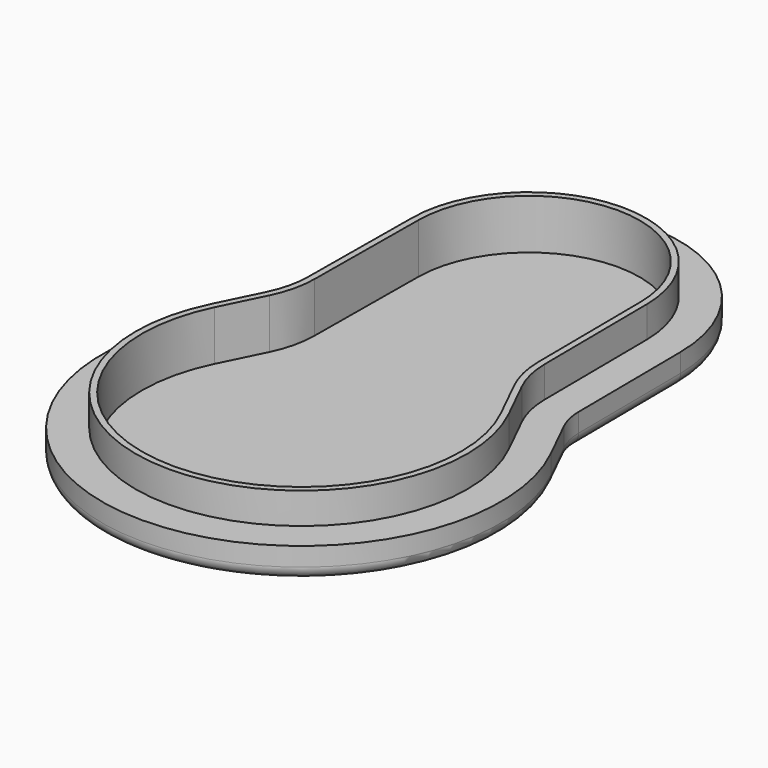
from build123d import *

# Parameters (mm, degrees)
F2_DEPTH = 4
F4_DEPTH = 1
F5_R     = 0.99999
F7_DEPTH = 1.5


# Not quite as in the source:
# - a fillet or chamfer is up to 0.001 mm smaller than in the source, because OpenCascade refuses the exact size


with BuildPart() as f2:
    # F1 (on face) → F2 (new body)
    with BuildSketch(Plane.XY):
        with BuildLine():
            ThreePointArc((-9.4849269336, 12.5314274341), (-9.6870039278, 10.8628934269), (-10.2555653995, 9.2812554476))
            Line((-10.2555653995, 9.2812554476), (-11.9329496797, 5.8732198956))
            ThreePointArc((-11.9329496797, 5.8732198956), (0, -13.3), (11.9329496797, 5.8732198956))
            Line((11.9329496797, 5.8732198956), (10.2555653995, 9.2812554476))
            ThreePointArc((10.2555653995, 9.2812554476), (9.6870039278, 10.8628934269), (9.4849269336, 12.5314274341))
            Line((9.4849269336, 12.5314274341), (9.3996809366, 22.8774486305))
            ThreePointArc((9.3996809366, 22.8774486305), (0, 32.2), (-9.3996809366, 22.8774486305))
            Line((-9.3996809366, 22.8774486305), (-9.4849269336, 12.5314274341))
        make_face()
        with BuildLine():
            ThreePointArc((-9.8069582687, 9.0604577072), (-9.2004926988, 10.7475382184), (-8.9849439051, 12.5273078261))
            Line((-8.9849439051, 12.5273078261), (-8.899697908, 22.8733290225))
            ThreePointArc((-8.899697908, 22.8733290225), (0, 31.7), (8.899697908, 22.8733290225))
            Line((8.899697908, 22.8733290225), (8.9849439051, 12.5273078261))
            ThreePointArc((8.9849439051, 12.5273078261), (9.2004926988, 10.7475382184), (9.8069582687, 9.0604577072))
            Line((9.8069582687, 9.0604577072), (11.4843425489, 5.6524221551))
            ThreePointArc((11.4843425489, 5.6524221551), (0, -12.8), (-11.4843425489, 5.6524221551))
            Line((-11.4843425489, 5.6524221551), (-9.8069582687, 9.0604577072))
        make_face(mode=Mode.SUBTRACT)
    extrude(amount=F2_DEPTH)

    # F3 (on face) + F0 (on Top) → F4 (join)
    with BuildSketch(Plane.XY):
        with BuildLine():
            ThreePointArc((12.6780439059, 10.473563246), (12.314164564, 11.4858115527), (12.1848352877, 12.5536733173))
            Line((12.1848352877, 12.5536733173), (12.0995892907, 22.8996945138))
            ThreePointArc((12.0995892907, 22.8996945138), (0, 34.9), (-12.0995892907, 22.8996945138))
            Line((-12.0995892907, 22.8996945138), (-12.1848352877, 12.5536733173))
            ThreePointArc((-12.1848352877, 12.5536733173), (-12.314164564, 11.4858115527), (-12.6780439059, 10.473563246))
            Line((-12.6780439059, 10.473563246), (-14.3554281861, 7.0655276939))
            ThreePointArc((-14.3554281861, 7.0655276939), (0, -16), (14.3554281861, 7.0655276939))
            Line((14.3554281861, 7.0655276939), (12.6780439059, 10.473563246))
        make_face()
        with BuildLine():
            ThreePointArc((-8.899697908, 22.8733290225), (0, 31.7), (8.899697908, 22.8733290225))
            Line((8.899697908, 22.8733290225), (8.9849439051, 12.5273078261))
            ThreePointArc((8.9849439051, 12.5273078261), (9.2004926988, 10.7475382184), (9.8069582687, 9.0604577072))
            Line((9.8069582687, 9.0604577072), (11.4843425489, 5.6524221551))
            ThreePointArc((11.4843425489, 5.6524221551), (0, -12.8), (-11.4843425489, 5.6524221551))
            Line((-11.4843425489, 5.6524221551), (-9.8069582687, 9.0604577072))
            ThreePointArc((-9.8069582687, 9.0604577072), (-9.2004926988, 10.7475382184), (-8.9849439051, 12.5273078261))
            Line((-8.9849439051, 12.5273078261), (-8.899697908, 22.8733290225))
        make_face(mode=Mode.SUBTRACT)
    with BuildSketch(Plane.XY):
        with BuildLine():
            Line((-9.8069582687, 9.0604577072), (-11.4843425489, 5.6524221551))
            ThreePointArc((-11.4843425489, 5.6524221551), (0, -12.8), (11.4843425489, 5.6524221551))
            Line((11.4843425489, 5.6524221551), (9.8069582687, 9.0604577072))
            ThreePointArc((9.8069582687, 9.0604577072), (9.2004926988, 10.7475382184), (8.9849439051, 12.5273078261))
            Line((8.9849439051, 12.5273078261), (8.899697908, 22.8733290225))
            ThreePointArc((8.899697908, 22.8733290225), (0, 31.7), (-8.899697908, 22.8733290225))
            Line((-8.899697908, 22.8733290225), (-8.9849439051, 12.5273078261))
            ThreePointArc((-8.9849439051, 12.5273078261), (-9.2004926988, 10.7475382184), (-9.8069582687, 9.0604577072))
        make_face()
    extrude(amount=-F4_DEPTH)

    # F5 (radius 1 in the source; OpenCascade refuses exactly that, so slightly less here)
    f5_edges = [f2.edges().sort_by_distance(p)[0] for p in [
        (0, -16, -1),
        (-13.516736, 8.769545, -1),
        (-12.314165, 11.485812, -1),
        (-12.142212, 17.726684, -1),
        (0, 34.9, -1),
        (12.142212, 17.726684, -1),
        (12.314165, 11.485812, -1),
        (13.516736, 8.769545, -1),
    ]]
    fillet(f5_edges, radius=F5_R)

    # F6 (on face) → F7 (join)
    with BuildSketch(Plane.XY):
        with BuildLine():
            ThreePointArc((-12.1848352877, 12.5536733173), (-12.314164564, 11.4858115527), (-12.6780439059, 10.473563246))
            Line((-12.6780439059, 10.473563246), (-14.3554281861, 7.0655276939))
            ThreePointArc((-14.3554281861, 7.0655276939), (0, -16), (14.3554281861, 7.0655276939))
            Line((14.3554281861, 7.0655276939), (12.6780439059, 10.473563246))
            ThreePointArc((12.6780439059, 10.473563246), (12.314164564, 11.4858115527), (12.1848352877, 12.5536733173))
            Line((12.1848352877, 12.5536733173), (12.0995892907, 22.8996945138))
            ThreePointArc((12.0995892907, 22.8996945138), (0, 34.9), (-12.0995892907, 22.8996945138))
            ThreePointArc((-12.0995892907, 22.8996945138), (-10.0273713078, 17.7092586924), (-12.1848352877, 12.5536733173))
        make_face()
        with BuildLine():
            ThreePointArc((-10.2555653995, 9.2812554476), (-9.6870039278, 10.8628934269), (-9.4849269336, 12.5314274341))
            Line((-9.4849269336, 12.5314274341), (-9.3996809366, 22.8774486305))
            ThreePointArc((-9.3996809366, 22.8774486305), (0, 32.2), (9.3996809366, 22.8774486305))
            Line((9.3996809366, 22.8774486305), (9.4849269336, 12.5314274341))
            ThreePointArc((9.4849269336, 12.5314274341), (9.6870039278, 10.8628934269), (10.2555653995, 9.2812554476))
            Line((10.2555653995, 9.2812554476), (11.9329496797, 5.8732198956))
            ThreePointArc((11.9329496797, 5.8732198956), (0, -13.3), (-11.9329496797, 5.8732198956))
            Line((-11.9329496797, 5.8732198956), (-10.2555653995, 9.2812554476))
        make_face(mode=Mode.SUBTRACT)
    extrude(amount=F7_DEPTH)


solid = f2.part
